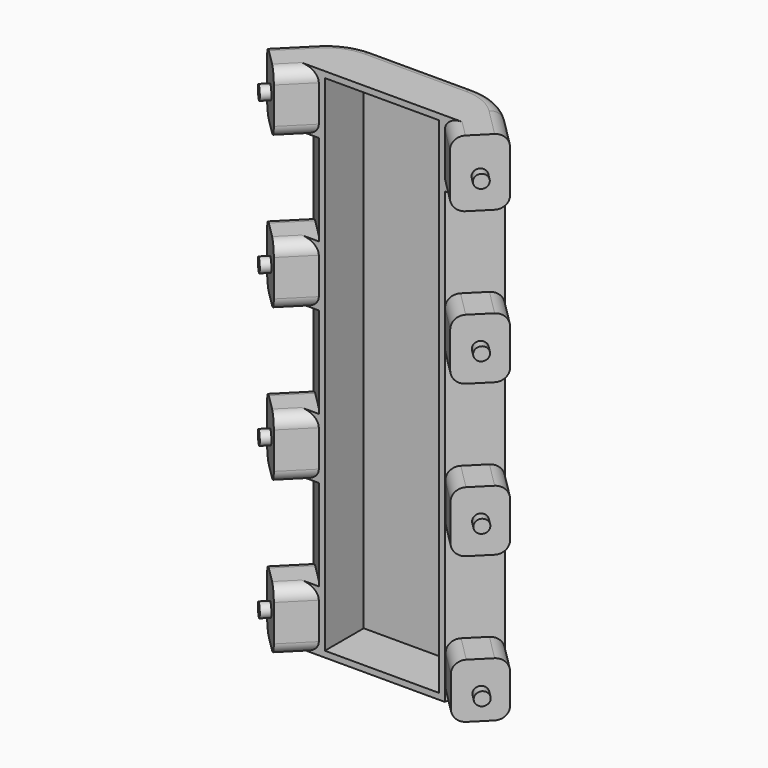
from build123d import *

# Parameters (mm, degrees)
F1_DEPTH  = 85
F2_R      = 10
F4_DEPTH  = 6
F5_R      = 2
F6_W      = 7.7781745931
F6_H      = 15
F7_DEPTH  = 6
F8_R      = 2
F6_R      = 1.1
F9_DEPTH  = 1.5
F3_R      = 1.1
F10_DEPTH = 1.5
F11_W     = 18.7703792453
F11_H     = 83
F12_DEPTH = 8


with BuildPart() as f1:
    # F0 (on Top) → F1 (new body)
    with BuildSketch(Plane.XY):
        Polygon((-20, 20), (-14.5, 14.5), (-10.3851896226, 18.6148103774), (0, 18.6148103774), (10.3851896226, 18.6148103774), (14.5, 14.5), (20, 20), (12.470660899, 27.529339101), (0, 27.529339101), (-12.470660899, 27.529339101), align=None)
    extrude(amount=F1_DEPTH)

    # F2
    f2_edges = [f1.edges().sort_by_distance(p)[0] for p in [
        (-12.470661, 27.529339, 42.5),
        (12.470661, 27.529339, 42.5),
    ]]
    fillet(f2_edges, radius=F2_R)

    # F3 (on face) → F4 (cut)
    with BuildSketch(Plane(origin=(0, 0, 0), x_dir=(0.7071067812, 0.7071067812, 0), z_dir=(0.7071067812, -0.7071067812, 0))):
        Polygon((28.2842712475, 59.0200200677), (28.2842712475, 74.0199925453), (20.5060966544, 74.0199925453), (20.5060966544, 0), (20.6173848753, 0), (20.6173848753, 9.0200751125), (28.2842712475, 9.0200751125), (28.2842712475, 24.0200475901), (20.5802888017, 24.0200475901), (20.5802888017, 34.0200475901), (28.2842712475, 34.0200475901), (28.2842712475, 49.0200200677), (20.543192728, 49.0200200677), (20.543192728, 59.0200200677), align=None)
    extrude(amount=-F4_DEPTH, mode=Mode.SUBTRACT)

    # F5
    f5_edges = [f1.edges().sort_by_distance(p)[0] for p in [
        (17.87868, 22.12132, 74.019993),
        (17.87868, 22.12132, 49.02002),
        (17.87868, 22.12132, 24.020048),
        (17.699797, 22.300203, 0),
        (12.457372, 16.700013, 0),
        (12.431141, 16.673782, 24.020048),
        (12.404911, 16.647551, 49.02002),
        (17.699797, 22.300203, 85),
        (12.442595, 16.557405, 85),
        (17.87868, 22.12132, 59.02002),
        (12.404911, 16.647551, 59.02002),
        (17.87868, 22.12132, 34.020048),
        (12.431141, 16.673782, 34.020048),
        (17.87868, 22.12132, 9.020075),
        (12.457372, 16.700013, 9.020075),
        (-17.699797, 22.300203, 0),
        (-17.699797, 22.300203, 85),
        (-12.15536, 26.768134, 0),
        (0, 27.529339, 0),
        (12.15536, 26.768134, 0),
        (-12.442595, 16.557405, 0),
        (-12.15536, 26.768134, 85),
        (0, 27.529339, 85),
        (-12.442595, 16.557405, 85),
        (12.15536, 26.768134, 85),
        (12.442595, 16.557405, 74.019993),
    ]]
    fillet(f5_edges, radius=F5_R)

    # F6 (on face) → F7 (cut)
    with BuildSketch(Plane(origin=(0, 0, 0), x_dir=(0.7071067812, -0.7071067812, 0), z_dir=(-0.7071067812, -0.7071067812, 0))):
        with Locations((-24.3951839509, 17.5)):
            Rectangle(F6_W, F6_H)
        with Locations((-24.3951839509, 42.5)):
            Rectangle(F6_W, F6_H)
        with Locations((-24.3951839509, 67.5)):
            Rectangle(F6_W, F6_H)
    extrude(amount=-F7_DEPTH, mode=Mode.SUBTRACT)

    # F8
    f8_edges = [f1.edges().sort_by_distance(p)[0] for p in [
        (-17.87868, 22.12132, 35),
        (-17.87868, 22.12132, 50),
        (-17.87868, 22.12132, 60),
        (-17.87868, 22.12132, 75),
        (-12.442595, 16.557405, 75),
        (-12.442595, 16.557405, 60),
        (-12.442595, 16.557405, 50),
        (-12.442595, 16.557405, 35),
        (-12.442595, 16.557405, 25),
        (-12.442595, 16.557405, 10),
        (-17.87868, 22.12132, 10),
        (-17.87868, 22.12132, 25),
    ]]
    fillet(f8_edges, radius=F8_R)

    # F6 (on face) → F9 (join)
    with BuildSketch(Plane(origin=(0, 0, 0), x_dir=(0.7071067812, -0.7071067812, 0), z_dir=(-0.7071067812, -0.7071067812, 0))):
        with Locations((-24.3951839509, 5)):
            Circle(F6_R)
        with Locations((-24.3951839509, 30)):
            Circle(F6_R)
        with Locations((-24.3951839509, 55)):
            Circle(F6_R)
        with Locations((-24.3951839509, 80)):
            Circle(F6_R)
    extrude(amount=F9_DEPTH)

    # F3 (on face) → F10 (join)
    with BuildSketch(Plane(origin=(0, 0, 0), x_dir=(0.7071067812, 0.7071067812, 0), z_dir=(0.7071067812, -0.7071067812, 0))):
        with Locations((24.3951839509, 79.0199925453)):
            Circle(F3_R)
        with Locations((24.4336626312, 54.0200221575)):
            Circle(F3_R)
        with Locations((24.4721413114, 29.0200517697)):
            Circle(F3_R)
        with Locations((24.5106199916, 4.0200813819)):
            Circle(F3_R)
    extrude(amount=F10_DEPTH)

    # F11 (on face) → F12 (cut)
    with BuildSketch(Plane.XZ.offset(-18.6148103774)):
        with Locations((0, 42.5)):
            Rectangle(F11_W, F11_H)
    extrude(amount=-F12_DEPTH, mode=Mode.SUBTRACT)


solid = f1.part
